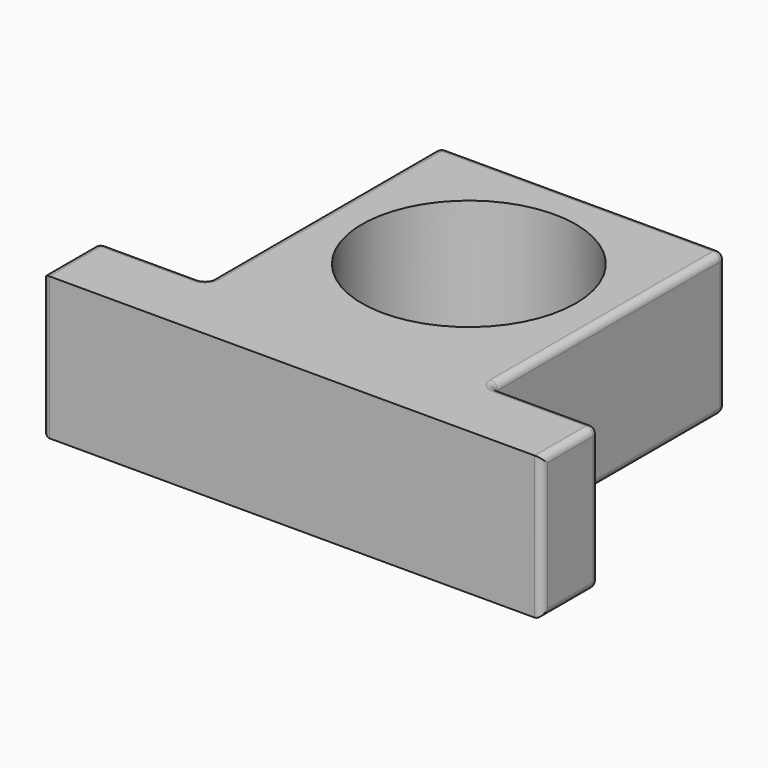
from build123d import *

# Parameters (mm, degrees)
F0_R     = 15
F0_W     = 15
F0_H     = 10
F1_DEPTH = 20
F2_F1_R  = 1
F2_F2_R  = 1
F3_R     = 1


with BuildPart() as f1:
    # F0 (on Top) → F1 (new body)
    with BuildSketch(Plane.XY):
        Polygon((-20, -25.5), (20, -25.5), (20, -15.5), (20, 25.5), (-20, 25.5), (-20, -15.5), align=None)
        with Locations((0, 5.5)):
            Circle(F0_R, mode=Mode.SUBTRACT)
        with Locations((-27.5, -20.5)):
            Rectangle(F0_W, F0_H)
        with Locations((27.5, -20.5)):
            Rectangle(F0_W, F0_H)
    extrude(amount=F1_DEPTH)

    # F2: fillet of radius 1 on 10 edges, made by hand

    # F2_f1
    f2_f1_edges = [f1.edges().sort_by_distance(p)[0] for p in [
        (-20, -15.5, 10),
        (20, -15.5, 10),
    ]]
    fillet(f2_f1_edges, radius=F2_F1_R)

    # F2_f2
    f2_f2_edges = [f1.edges().sort_by_distance(p)[0] for p in [
        (-20, 25.5, 10),
        (-20, 5.5, 0),
        (-20, 5.5, 20),
        (20, 25.5, 10),
        (0, 25.5, 0),
        (0, 25.5, 20),
        (20, 5.5, 0),
        (20, 5.5, 20),
        (20.2928932188, -15.2071067812, 20),
        (20.2928932188, -15.2071067812, 0),
        (-20.2928932188, -15.2071067812, 20),
        (-20.2928932188, -15.2071067812, 0),
    ]]
    fillet(f2_f2_edges, radius=F2_F2_R)

    # F3
    f3_edges = [f1.edges().sort_by_distance(p)[0] for p in [
        (21, -15.5, 10),
        (28, -15.5, 1),
        (28, -15.5, 19),
        (35, -15.5, 10),
        (35, -15.792893, 0.292893),
        (35, -15.792893, 19.707107),
        (35, -21, 0),
        (35, -21, 20),
        (35, -25.5, 10),
        (-21, -15.5, 10),
        (-28, -15.5, 1),
        (-28, -15.5, 19),
        (-35, -15.5, 10),
        (-35, -15.792893, 0.292893),
        (-35, -15.792893, 19.707107),
        (-35, -21, 0),
        (-35, -21, 20),
        (-35, -25.5, 10),
    ]]
    fillet(f3_edges, radius=F3_R)


solid = f1.part
